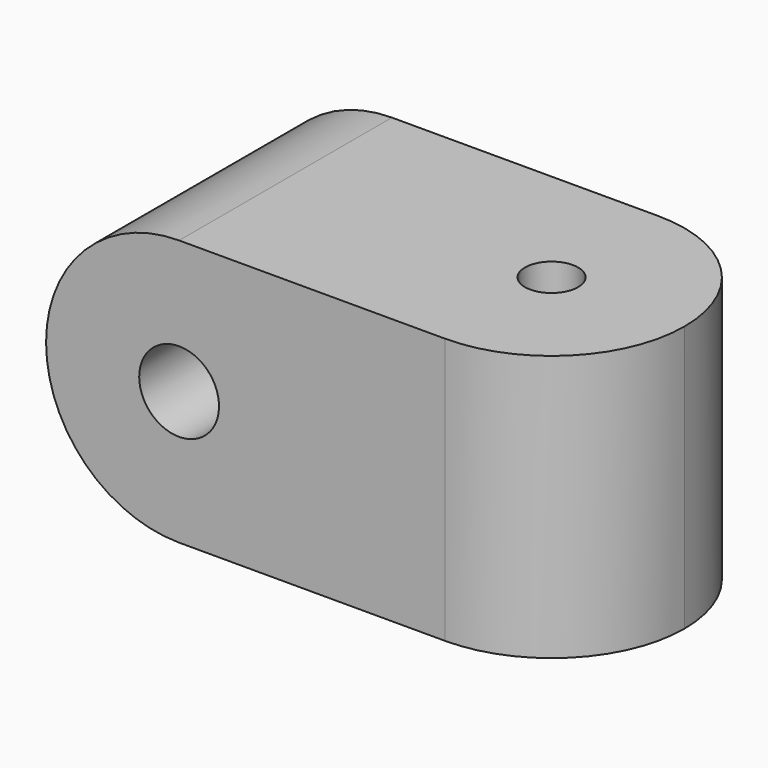
from build123d import *

# Parameters (mm, degrees)
F0_W     = 39.9999970493
F0_H     = 20
F1_DEPTH = 20
F3_D     = 4
F5_D     = 6
F6_R     = 9.99999
F7_R     = 9.99999


# Not quite as in the source:
# - a fillet or chamfer is up to 0.001 mm smaller than in the source, because OpenCascade refuses the exact size


with BuildPart() as f1:
    # F0 (on Top) → F1 (new body)
    with BuildSketch(Plane.XY):
        with Locations((19.9999985246, 10)):
            Rectangle(F0_W, F0_H)
    extrude(amount=F1_DEPTH)

    # F3 (through all)
    with Locations(Plane.XY.offset(20)):
        with Locations((30.0000011921, 10)):
            Hole(F3_D / 2)

    # F5 (through all)
    with Locations(Plane.XZ):
        with Locations((10, 10)):
            Hole(F5_D / 2)

    # F6 (radius 10 in the source; OpenCascade refuses exactly that, so slightly less here)
    f6_edges = [f1.edges().sort_by_distance(p)[0] for p in [
        (39.999997, 0, 10),
        (39.999997, 20, 10),
    ]]
    fillet(f6_edges, radius=F6_R)

    # F7 (radius 10 in the source; OpenCascade refuses exactly that, so slightly less here)
    f7_edges = [f1.edges().sort_by_distance(p)[0] for p in [
        (0, 10, 0),
        (0, 10, 20),
    ]]
    fillet(f7_edges, radius=F7_R)


solid = f1.part
